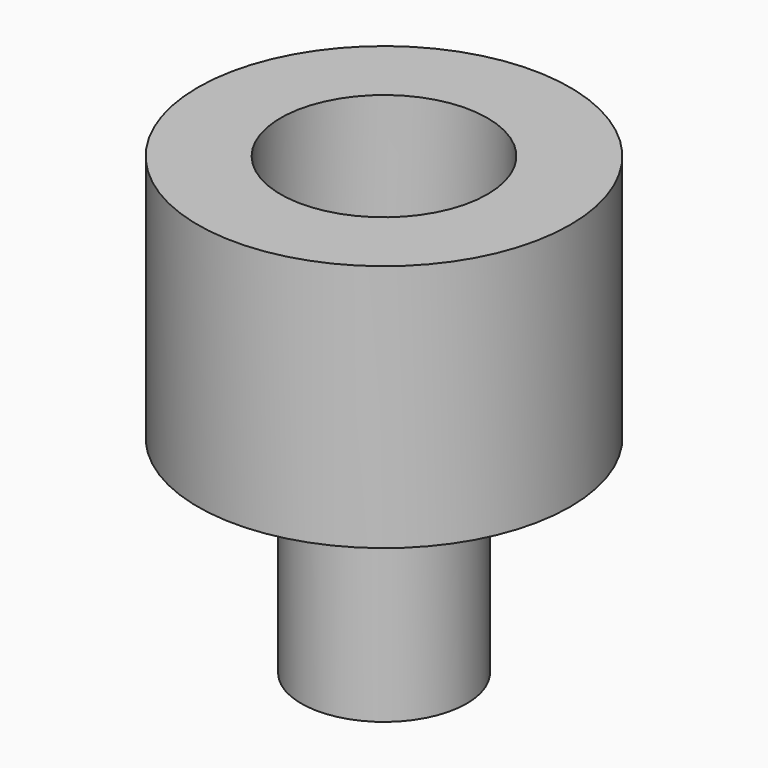
from build123d import *

# Parameters (mm, degrees)
F0_R     = 4.5
F1_DEPTH = 6
F2_T     = -2
F3_R     = 2
F4_DEPTH = 5
F5_T     = 1
F6_R     = 1
F7_DEPTH = 12.5


# Not quite as in the source:
# - a shell that OpenCascade refuses in one call is made with other operations: the cavity is built on its own and cut out


with BuildPart() as f1:
    # F0 (on Top) → F1 (new body)
    with BuildSketch(Plane.XY):
        Circle(F0_R)
    extrude(amount=F1_DEPTH)

    # F2
    f2_openings = [f1.faces().sort_by_distance(p)[0] for p in [
        (0, 0, 6),
    ]]
    offset(amount=F2_T, openings=f2_openings)

    # F3 (on face) → F4 (join)
    with BuildSketch(Plane(origin=(0, 0, 0), x_dir=(1, 0, 0), z_dir=(0, 0, -1))):
        Circle(F3_R)
    extrude(amount=F4_DEPTH)

    # F5: shell of thickness 1, made by hand


with BuildPart() as f5_core1:
    # F5_t2: copy of F1
    add(f1.part)

    # the walls: a layer under each face that stays
    f5_faces = [f5_core1.faces().sort_by_distance(p)[0] for p in [
        (-4.5, 0, 3),
        (-3, -3, 0),
        (-3, -3, 6),
        (-2, 0, -2.5),
        (-2.5, 0, 4),
        (0, 0, 2),
    ]]
    thicken(f5_faces, amount=-F5_T, mode=Mode.SUBTRACT)

    # F5_s3 → F5_t4 (revolve, cut)
    with BuildSketch(Plane.XZ):
        Polygon((2.01, -0.01), (2, 1), (1, 1), (1, 0), align=None)
    revolve(axis=Axis((0, 0, 0), (0, 0, -1)), mode=Mode.SUBTRACT)

    # F5_s5 → F5_t6 (revolve, cut)
    with BuildSketch(Plane.XZ):
        Polygon((2.49, 2.01), (3.5, 2), (3.5, 1), (2.5, 1), align=None)
    revolve(axis=Axis((0, 0, 2), (0, 0, -1)), mode=Mode.SUBTRACT)


with BuildPart() as f1_1:
    add(f1.part)

    # what is left inside the walls is the cavity
    f5_cavity = [f5_core1.part.solids().sort_by_distance(p)[0] for p in [
        (-0.99, 0, -1),
    ]]
    add(f5_cavity, mode=Mode.SUBTRACT)

    # F6 (on face) → F7 (cut, symmetric)
    with BuildSketch(Plane(origin=(0, 0, 0), x_dir=(1, 0, 0), z_dir=(0, 0, -1))):
        Circle(F6_R)
    extrude(amount=F7_DEPTH, both=True, mode=Mode.SUBTRACT)


solid = f1_1.part
